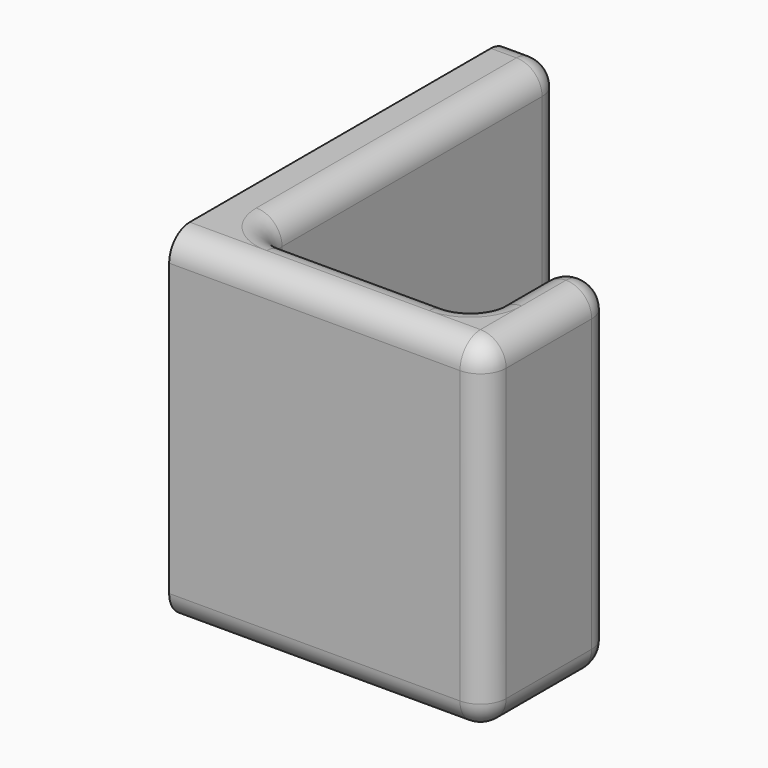
from build123d import *

# Parameters (mm, degrees)
F1_DEPTH = 20
F2_R     = 1.49999


# Not quite as in the source:
# - a fillet or chamfer is up to 0.001 mm smaller than in the source, because OpenCascade refuses the exact size


with BuildPart() as f1:
    # F0 (on Top) → F1 (new body)
    with BuildSketch(Plane.XY):
        with BuildLine():
            Line((1.5, 25), (0, 25))
            Line((0, 25), (0, 0))
            Line((0, 0), (17, 0))
            ThreePointArc((17, 0), (18.0606601718, 0.4393398282), (18.5, 1.5))
            Line((18.5, 1.5), (18.5, 7.75))
            ThreePointArc((18.5, 7.75), (18.0606601718, 8.8106601718), (17, 9.25))
            ThreePointArc((17, 9.25), (15.9393398282, 8.8106601718), (15.5, 7.75))
            Line((15.5, 7.75), (15.5, 4.5))
            ThreePointArc((15.5, 4.5), (15.0606601718, 3.4393398282), (14, 3))
            Line((14, 3), (4.5, 3))
            ThreePointArc((4.5, 3), (3.4393398282, 3.4393398282), (3, 4.5))
            Line((3, 4.5), (3, 23.5))
            ThreePointArc((3, 23.5), (2.5606601718, 24.5606601718), (1.5, 25))
        make_face()
    extrude(amount=F1_DEPTH)

    # F2 (radius 1.5 in the source; OpenCascade refuses exactly that, so slightly less here)
    f2_edges = [f1.edges().sort_by_distance(p)[0] for p in [
        (3, 14, 20),
        (9.25, 3, 0),
    ]]
    fillet(f2_edges, radius=F2_R)


solid = f1.part
